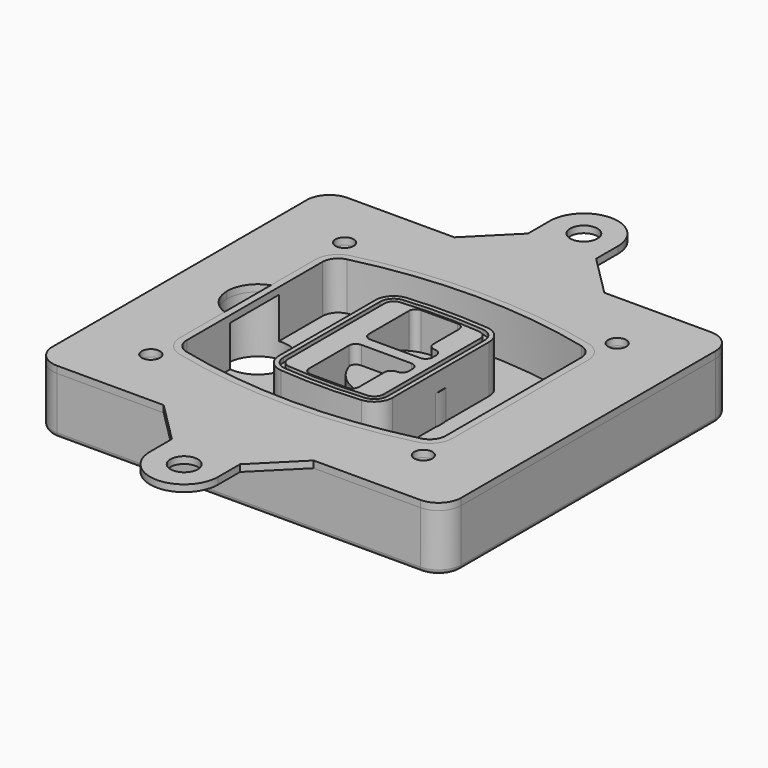
from build123d import *

# Parameters (mm, degrees)
F0_R      = 4
F1_DEPTH  = 25
F2_DEPTH  = 3
F3_DEPTH  = 18
F5_DEPTH  = 21
F6_DEPTH  = 2
F8_DEPTH  = 20
F9_DEPTH  = 16
F10_DEPTH = 25
F7_R      = 6
F7_R_2    = 4
F11_DEPTH = 6
F13_DEPTH = 9
F15_R     = 2
F16_R     = 6
F16_R_2   = 4
F17_DEPTH = 3


# Not quite as in the source:
# - a feature of the source that left no trace in its solid (it failed there, or was rolled back) is left out
# - a feature names something its author has since deleted; it is built from what else it names


with BuildPart() as f1:
    # F0 (on Top) → F1 (new body)
    with BuildSketch(Plane.XY):
        with BuildLine():
            ThreePointArc((-90, -70), (-87.0710678119, -77.0710678119), (-80, -80))
            Line((-80, -80), (80, -80))
            ThreePointArc((80, -80), (87.0710678119, -77.0710678119), (90, -70))
            Line((90, -70), (90, 70))
            ThreePointArc((90, 70), (87.0710678119, 77.0710678119), (80, 80))
            Line((80, 80), (-80, 80))
            ThreePointArc((-80, 80), (-87.0710678119, 77.0710678119), (-90, 70))
            Line((-90, 70), (-90, -70))
        make_face()
        with Locations((-60, -53.3333333333)):
            Circle(F0_R, mode=Mode.SUBTRACT)
        with Locations((60, -53.3333333333)):
            Circle(F0_R, mode=Mode.SUBTRACT)
        with Locations((-60, 53.3333333333)):
            Circle(F0_R, mode=Mode.SUBTRACT)
        with BuildLine():
            ThreePointArc((-64, 37.2990447398), (-61.0143011354, 45.9411029726), (-53.3306899286, 50.8970778549))
            ThreePointArc((-53.3306899286, 50.8970778549), (0, 57.3333333333), (53.3306899286, 50.8970778549))
            ThreePointArc((53.3306899286, 50.8970778549), (61.0143011354, 45.9411029726), (64, 37.2990447398))
            Line((64, 37.2990447398), (64, -37.2990447398))
            ThreePointArc((64, -37.2990447398), (61.0143011354, -45.9411029726), (53.3306899286, -50.8970778549))
            ThreePointArc((53.3306899286, -50.8970778549), (0, -57.3333333333), (-53.3306899286, -50.8970778549))
            ThreePointArc((-53.3306899286, -50.8970778549), (-61.0143011354, -45.9411029726), (-64, -37.2990447398))
            Line((-64, -37.2990447398), (-64, 37.2990447398))
        make_face(mode=Mode.SUBTRACT)
        with Locations((60, 53.3333333333)):
            Circle(F0_R, mode=Mode.SUBTRACT)
        with BuildLine():
            ThreePointArc((53.3306899286, 50.8970778549), (0, 57.3333333333), (-53.3306899286, 50.8970778549))
            ThreePointArc((-53.3306899286, 50.8970778549), (-61.0143011354, 45.9411029726), (-64, 37.2990447398))
            Line((-64, 37.2990447398), (-64, -37.2990447398))
            ThreePointArc((-64, -37.2990447398), (-61.0143011354, -45.9411029726), (-53.3306899286, -50.8970778549))
            ThreePointArc((-53.3306899286, -50.8970778549), (0, -57.3333333333), (53.3306899286, -50.8970778549))
            ThreePointArc((53.3306899286, -50.8970778549), (61.0143011354, -45.9411029726), (64, -37.2990447398))
            Line((64, -37.2990447398), (64, 37.2990447398))
            ThreePointArc((64, 37.2990447398), (61.0143011354, 45.9411029726), (53.3306899286, 50.8970778549))
        make_face()
        with BuildLine():
            Line((-60, -37.2990447398), (-60, 37.2990447398))
            ThreePointArc((-60, 37.2990447398), (-57.8673579538, 43.4719434775), (-52.3790642347, 47.0119255363))
            ThreePointArc((-52.3790642347, 47.0119255363), (0, 53.3333333333), (52.3790642347, 47.0119255363))
            ThreePointArc((52.3790642347, 47.0119255363), (57.8673579538, 43.4719434775), (60, 37.2990447398))
            Line((60, 37.2990447398), (60, -37.2990447398))
            ThreePointArc((60, -37.2990447398), (57.8673579538, -43.4719434775), (52.3790642347, -47.0119255363))
            ThreePointArc((52.3790642347, -47.0119255363), (0, -53.3333333333), (-52.3790642347, -47.0119255363))
            ThreePointArc((-52.3790642347, -47.0119255363), (-57.8673579538, -43.4719434775), (-60, -37.2990447398))
        make_face(mode=Mode.SUBTRACT)
        with BuildLine():
            ThreePointArc((-52.3790642347, 47.0119255363), (-57.8673579538, 43.4719434775), (-60, 37.2990447398))
            Line((-60, 37.2990447398), (-60, -37.2990447398))
            ThreePointArc((-60, -37.2990447398), (-57.8673579538, -43.4719434775), (-52.3790642347, -47.0119255363))
            ThreePointArc((-52.3790642347, -47.0119255363), (0, -53.3333333333), (52.3790642347, -47.0119255363))
            ThreePointArc((52.3790642347, -47.0119255363), (57.8673579538, -43.4719434775), (60, -37.2990447398))
            Line((60, -37.2990447398), (60, 37.2990447398))
            ThreePointArc((60, 37.2990447398), (57.8673579538, 43.4719434775), (52.3790642347, 47.0119255363))
            ThreePointArc((52.3790642347, 47.0119255363), (0, 53.3333333333), (-52.3790642347, 47.0119255363))
        make_face()
        with BuildLine():
            ThreePointArc((51.6653449643, 44.0980612973), (55.5071505677, 41.6200738562), (57, 37.2990447398))
            Line((57, 37.2990447398), (57, -37.2990447398))
            ThreePointArc((57, -37.2990447398), (55.5071505677, -41.6200738562), (51.6653449643, -44.0980612973))
            ThreePointArc((51.6653449643, -44.0980612973), (0, -50.3333333333), (-51.6653449643, -44.0980612973))
            ThreePointArc((-51.6653449643, -44.0980612973), (-55.5071505677, -41.6200738562), (-57, -37.2990447398))
            Line((-57, -37.2990447398), (-57, 37.2990447398))
            ThreePointArc((-57, 37.2990447398), (-55.5071505677, 41.6200738562), (-51.6653449643, 44.0980612973))
            ThreePointArc((-51.6653449643, 44.0980612973), (0, 50.3333333333), (51.6653449643, 44.0980612973))
        make_face(mode=Mode.SUBTRACT)
        with BuildLine():
            Line((57, -37.2990447398), (57, 37.2990447398))
            ThreePointArc((57, 37.2990447398), (55.5071505677, 41.6200738562), (51.6653449643, 44.0980612973))
            ThreePointArc((51.6653449643, 44.0980612973), (0, 50.3333333333), (-51.6653449643, 44.0980612973))
            ThreePointArc((-51.6653449643, 44.0980612973), (-55.5071505677, 41.6200738562), (-57, 37.2990447398))
            Line((-57, 37.2990447398), (-57, -37.2990447398))
            ThreePointArc((-57, -37.2990447398), (-55.5071505677, -41.6200738562), (-51.6653449643, -44.0980612973))
            ThreePointArc((-51.6653449643, -44.0980612973), (0, -50.3333333333), (51.6653449643, -44.0980612973))
            ThreePointArc((51.6653449643, -44.0980612973), (55.5071505677, -41.6200738562), (57, -37.2990447398))
        make_face()
    extrude(amount=-F1_DEPTH)

    # F0 (on Top) → F2 (join)
    with BuildSketch(Plane.XY):
        with BuildLine():
            ThreePointArc((-52.3790642347, 47.0119255363), (-57.8673579538, 43.4719434775), (-60, 37.2990447398))
            Line((-60, 37.2990447398), (-60, -37.2990447398))
            ThreePointArc((-60, -37.2990447398), (-57.8673579538, -43.4719434775), (-52.3790642347, -47.0119255363))
            ThreePointArc((-52.3790642347, -47.0119255363), (0, -53.3333333333), (52.3790642347, -47.0119255363))
            ThreePointArc((52.3790642347, -47.0119255363), (57.8673579538, -43.4719434775), (60, -37.2990447398))
            Line((60, -37.2990447398), (60, 37.2990447398))
            ThreePointArc((60, 37.2990447398), (57.8673579538, 43.4719434775), (52.3790642347, 47.0119255363))
            ThreePointArc((52.3790642347, 47.0119255363), (0, 53.3333333333), (-52.3790642347, 47.0119255363))
        make_face()
        with BuildLine():
            ThreePointArc((51.6653449643, 44.0980612973), (55.5071505677, 41.6200738562), (57, 37.2990447398))
            Line((57, 37.2990447398), (57, -37.2990447398))
            ThreePointArc((57, -37.2990447398), (55.5071505677, -41.6200738562), (51.6653449643, -44.0980612973))
            ThreePointArc((51.6653449643, -44.0980612973), (0, -50.3333333333), (-51.6653449643, -44.0980612973))
            ThreePointArc((-51.6653449643, -44.0980612973), (-55.5071505677, -41.6200738562), (-57, -37.2990447398))
            Line((-57, -37.2990447398), (-57, 37.2990447398))
            ThreePointArc((-57, 37.2990447398), (-55.5071505677, 41.6200738562), (-51.6653449643, 44.0980612973))
            ThreePointArc((-51.6653449643, 44.0980612973), (0, 50.3333333333), (51.6653449643, 44.0980612973))
        make_face(mode=Mode.SUBTRACT)
    extrude(amount=F2_DEPTH)

    # F0 (on Top) → F3 (cut)
    with BuildSketch(Plane.XY):
        with BuildLine():
            Line((57, -37.2990447398), (57, 37.2990447398))
            ThreePointArc((57, 37.2990447398), (55.5071505677, 41.6200738562), (51.6653449643, 44.0980612973))
            ThreePointArc((51.6653449643, 44.0980612973), (0, 50.3333333333), (-51.6653449643, 44.0980612973))
            ThreePointArc((-51.6653449643, 44.0980612973), (-55.5071505677, 41.6200738562), (-57, 37.2990447398))
            Line((-57, 37.2990447398), (-57, -37.2990447398))
            ThreePointArc((-57, -37.2990447398), (-55.5071505677, -41.6200738562), (-51.6653449643, -44.0980612973))
            ThreePointArc((-51.6653449643, -44.0980612973), (0, -50.3333333333), (51.6653449643, -44.0980612973))
            ThreePointArc((51.6653449643, -44.0980612973), (55.5071505677, -41.6200738562), (57, -37.2990447398))
        make_face()
    extrude(amount=-F3_DEPTH, mode=Mode.SUBTRACT)

    # F4 (on face) → F5 (join, through all)
    with BuildSketch(Plane.XY.offset(3)):
        with BuildLine():
            ThreePointArc((-25, -26.587695628), (-22.8992979869, -31.9912392117), (-17.7004291845, -34.5569740744))
            ThreePointArc((-17.7004291845, -34.5569740744), (0, -35.3333333333), (17.7004291845, -34.5569740744))
            ThreePointArc((17.7004291845, -34.5569740744), (22.8992979869, -31.9912392117), (25, -26.587695628))
            Line((25, -26.587695628), (25, 26.587695628))
            ThreePointArc((25, 26.587695628), (22.8992979869, 31.9912392117), (17.7004291845, 34.5569740744))
            ThreePointArc((17.7004291845, 34.5569740744), (0, 35.3333333333), (-17.7004291845, 34.5569740744))
            ThreePointArc((-17.7004291845, 34.5569740744), (-22.8992979869, 31.9912392117), (-25, 26.587695628))
            Line((-25, 26.587695628), (-25, -26.587695628))
        make_face()
        with BuildLine():
            ThreePointArc((17.5253218884, 32.5646544628), (21.4244734902, 30.6403533158), (23, 26.587695628))
            Line((23, 26.587695628), (23, -26.587695628))
            ThreePointArc((23, -26.587695628), (21.4244734902, -30.6403533158), (17.5253218884, -32.5646544628))
            ThreePointArc((17.5253218884, -32.5646544628), (0, -33.3333333333), (-17.5253218884, -32.5646544628))
            ThreePointArc((-17.5253218884, -32.5646544628), (-21.4244734902, -30.6403533158), (-23, -26.587695628))
            Line((-23, -26.587695628), (-23, 26.587695628))
            ThreePointArc((-23, 26.587695628), (-21.4244734902, 30.6403533158), (-17.5253218884, 32.5646544628))
            ThreePointArc((-17.5253218884, 32.5646544628), (0, 33.3333333333), (17.5253218884, 32.5646544628))
        make_face(mode=Mode.SUBTRACT)
        with BuildLine():
            Line((23, -26.587695628), (23, 26.587695628))
            ThreePointArc((23, 26.587695628), (21.4244734902, 30.6403533158), (17.5253218884, 32.5646544628))
            ThreePointArc((17.5253218884, 32.5646544628), (0, 33.3333333333), (-17.5253218884, 32.5646544628))
            ThreePointArc((-17.5253218884, 32.5646544628), (-21.4244734902, 30.6403533158), (-23, 26.587695628))
            Line((-23, 26.587695628), (-23, -26.587695628))
            ThreePointArc((-23, -26.587695628), (-21.4244734902, -30.6403533158), (-17.5253218884, -32.5646544628))
            ThreePointArc((-17.5253218884, -32.5646544628), (0, -33.3333333333), (17.5253218884, -32.5646544628))
            ThreePointArc((17.5253218884, -32.5646544628), (21.4244734902, -30.6403533158), (23, -26.587695628))
        make_face()
        with BuildLine():
            ThreePointArc((17.3502145923, 30.5723348512), (19.9496489934, 29.2894674198), (21, 26.587695628))
            Line((21, 26.587695628), (21, -26.587695628))
            ThreePointArc((21, -26.587695628), (19.9496489934, -29.2894674198), (17.3502145923, -30.5723348512))
            ThreePointArc((17.3502145923, -30.5723348512), (0, -31.3333333333), (-17.3502145923, -30.5723348512))
            ThreePointArc((-17.3502145923, -30.5723348512), (-19.9496489934, -29.2894674198), (-21, -26.587695628))
            Line((-21, -26.587695628), (-21, 26.587695628))
            ThreePointArc((-21, 26.587695628), (-19.9496489934, 29.2894674198), (-17.3502145923, 30.5723348512))
            ThreePointArc((-17.3502145923, 30.5723348512), (0, 31.3333333333), (17.3502145923, 30.5723348512))
        make_face(mode=Mode.SUBTRACT)
        with BuildLine():
            Line((21, -26.587695628), (21, 26.587695628))
            ThreePointArc((21, 26.587695628), (19.9496489934, 29.2894674198), (17.3502145923, 30.5723348512))
            ThreePointArc((17.3502145923, 30.5723348512), (0, 31.3333333333), (-17.3502145923, 30.5723348512))
            ThreePointArc((-17.3502145923, 30.5723348512), (-19.9496489934, 29.2894674198), (-21, 26.587695628))
            Line((-21, 26.587695628), (-21, -26.587695628))
            ThreePointArc((-21, -26.587695628), (-19.9496489934, -29.2894674198), (-17.3502145923, -30.5723348512))
            ThreePointArc((-17.3502145923, -30.5723348512), (0, -31.3333333333), (17.3502145923, -30.5723348512))
            ThreePointArc((17.3502145923, -30.5723348512), (19.9496489934, -29.2894674198), (21, -26.587695628))
        make_face()
        with BuildLine():
            Line((-8, -2.5), (14, -2.5))
            ThreePointArc((14, -2.5), (16.1213203436, -3.3786796564), (17, -5.5))
            Line((17, -5.5), (17, -7.5))
            ThreePointArc((17, -7.5), (16.1213203436, -9.6213203436), (14, -10.5))
            ThreePointArc((14, -10.5), (11.8786796564, -11.3786796564), (11, -13.5))
            Line((11, -13.5), (11, -27.5))
            ThreePointArc((11, -27.5), (10.1213203436, -29.6213203436), (8, -30.5))
            Line((8, -30.5), (-8, -30.5))
            ThreePointArc((-8, -30.5), (-10.1213203436, -29.6213203436), (-11, -27.5))
            Line((-11, -27.5), (-11, -5.5))
            ThreePointArc((-11, -5.5), (-10.1213203436, -3.3786796564), (-8, -2.5))
        make_face(mode=Mode.SUBTRACT)
        with BuildLine():
            ThreePointArc((-8, 2.5), (-10.1213203436, 3.3786796564), (-11, 5.5))
            Line((-11, 5.5), (-11, 27.5))
            ThreePointArc((-11, 27.5), (-10.1213203436, 29.6213203436), (-8, 30.5))
            Line((-8, 30.5), (8, 30.5))
            ThreePointArc((8, 30.5), (10.1213203436, 29.6213203436), (11, 27.5))
            Line((11, 27.5), (11, 13.5))
            ThreePointArc((11, 13.5), (11.8786796564, 11.3786796564), (14, 10.5))
            ThreePointArc((14, 10.5), (16.1213203436, 9.6213203436), (17, 7.5))
            Line((17, 7.5), (17, 5.5))
            ThreePointArc((17, 5.5), (16.1213203436, 3.3786796564), (14, 2.5))
            Line((14, 2.5), (-8, 2.5))
        make_face(mode=Mode.SUBTRACT)
    extrude(amount=-F5_DEPTH)

    # F4 (on face) → F6 (cut)
    with BuildSketch(Plane.XY.offset(3)):
        with BuildLine():
            Line((23, -26.587695628), (23, 26.587695628))
            ThreePointArc((23, 26.587695628), (21.4244734902, 30.6403533158), (17.5253218884, 32.5646544628))
            ThreePointArc((17.5253218884, 32.5646544628), (0, 33.3333333333), (-17.5253218884, 32.5646544628))
            ThreePointArc((-17.5253218884, 32.5646544628), (-21.4244734902, 30.6403533158), (-23, 26.587695628))
            Line((-23, 26.587695628), (-23, -26.587695628))
            ThreePointArc((-23, -26.587695628), (-21.4244734902, -30.6403533158), (-17.5253218884, -32.5646544628))
            ThreePointArc((-17.5253218884, -32.5646544628), (0, -33.3333333333), (17.5253218884, -32.5646544628))
            ThreePointArc((17.5253218884, -32.5646544628), (21.4244734902, -30.6403533158), (23, -26.587695628))
        make_face()
        with BuildLine():
            ThreePointArc((17.3502145923, 30.5723348512), (19.9496489934, 29.2894674198), (21, 26.587695628))
            Line((21, 26.587695628), (21, -26.587695628))
            ThreePointArc((21, -26.587695628), (19.9496489934, -29.2894674198), (17.3502145923, -30.5723348512))
            ThreePointArc((17.3502145923, -30.5723348512), (0, -31.3333333333), (-17.3502145923, -30.5723348512))
            ThreePointArc((-17.3502145923, -30.5723348512), (-19.9496489934, -29.2894674198), (-21, -26.587695628))
            Line((-21, -26.587695628), (-21, 26.587695628))
            ThreePointArc((-21, 26.587695628), (-19.9496489934, 29.2894674198), (-17.3502145923, 30.5723348512))
            ThreePointArc((-17.3502145923, 30.5723348512), (0, 31.3333333333), (17.3502145923, 30.5723348512))
        make_face(mode=Mode.SUBTRACT)
    extrude(amount=-F6_DEPTH, mode=Mode.SUBTRACT)

    # F7 (on face) → F8 (join)
    with BuildSketch(Plane(origin=(0, 0, -25), x_dir=(1, 0, 0), z_dir=(0, 0, -1))):
        with BuildLine():
            ThreePointArc((-6.71157564, 0), (6.7567035675, 13.4682792075), (20.224982775, 0))
            Line((20.224982775, 0), (25.224982775, 0))
            ThreePointArc((25.224982775, 0), (6.7567035675, 18.4682792075), (-11.71157564, 0))
            Line((-11.71157564, 0), (-6.71157564, 0))
        make_face()
        with BuildLine():
            Line((-6.71157564, 0), (20.224982775, 0))
            ThreePointArc((20.224982775, 0), (6.7567035675, 13.4682792075), (-6.71157564, 0))
        make_face()
        with BuildLine():
            ThreePointArc((-6.71157564, 0), (6.7567035675, -13.4682792075), (20.224982775, 0))
            Line((20.224982775, 0), (-6.71157564, 0))
        make_face()
        with BuildLine():
            Line((25.224982775, 0), (20.224982775, 0))
            ThreePointArc((20.224982775, 0), (6.7567035675, -13.4682792075), (-6.71157564, 0))
            Line((-6.71157564, 0), (-11.71157564, 0))
            ThreePointArc((-11.71157564, 0), (6.7567035675, -18.4682792075), (25.224982775, 0))
        make_face()
    extrude(amount=-F8_DEPTH)

    # F7 (on face) → F9 (cut)
    with BuildSketch(Plane(origin=(0, 0, -25), x_dir=(1, 0, 0), z_dir=(0, 0, -1))):
        with BuildLine():
            Line((-6.71157564, 0), (20.224982775, 0))
            ThreePointArc((20.224982775, 0), (6.7567035675, 13.4682792075), (-6.71157564, 0))
        make_face()
        with BuildLine():
            ThreePointArc((-6.71157564, 0), (6.7567035675, -13.4682792075), (20.224982775, 0))
            Line((20.224982775, 0), (-6.71157564, 0))
        make_face()
    extrude(amount=-F9_DEPTH, mode=Mode.SUBTRACT)

    # F7 (on face) → F10 (cut)
    with BuildSketch(Plane(origin=(0, 0, -25), x_dir=(1, 0, 0), z_dir=(0, 0, -1))):
        with BuildLine():
            Line((-69.0318229325, 0), (-42.0952645175, 0))
            ThreePointArc((-42.0952645175, 0), (-55.563543725, 13.4682792075), (-69.0318229325, 0))
        make_face()
        with BuildLine():
            ThreePointArc((-69.0318229325, 0), (-55.563543725, -13.4682792075), (-42.0952645175, 0))
            Line((-42.0952645175, 0), (-69.0318229325, 0))
        make_face()
    extrude(amount=-F10_DEPTH, mode=Mode.SUBTRACT)

    # F7 (on face) → F11 (cut)
    with BuildSketch(Plane(origin=(0, 0, -25), x_dir=(1, 0, 0), z_dir=(0, 0, -1))):
        with Locations((60, -53.3333333333)):
            Circle(F7_R)
        with Locations((60, -53.3333333333)):
            Circle(F7_R_2, mode=Mode.SUBTRACT)
        with Locations((-60, -53.3333333333)):
            Circle(F7_R)
        with Locations((-60, -53.3333333333)):
            Circle(F7_R_2, mode=Mode.SUBTRACT)
        with Locations((-60, 53.3333333333)):
            Circle(F7_R)
        with Locations((-60, 53.3333333333)):
            Circle(F7_R_2, mode=Mode.SUBTRACT)
        with Locations((60, 53.3333333333)):
            Circle(F7_R)
        with Locations((60, 53.3333333333)):
            Circle(F7_R_2, mode=Mode.SUBTRACT)
    extrude(amount=-F11_DEPTH, mode=Mode.SUBTRACT)

    # F12 (on face) → F13 (cut, through all)
    with BuildSketch(Plane(origin=(0, 0, -9), x_dir=(1, 0, 0), z_dir=(0, 0, -1))):
        with BuildLine():
            ThreePointArc((20.224982775, 0), (20.1663399806, 1.2554664788), (19.9909222755, 2.5))
            Line((19.9909222755, 2.5), (14, 2.5))
            ThreePointArc((14, 2.5), (16.1213203436, 3.3786796564), (17, 5.5))
            Line((17, 5.5), (17, 7.5))
            ThreePointArc((17, 7.5), (16.1213203436, 9.6213203436), (14, 10.5))
            ThreePointArc((14, 10.5), (12.1627255951, 11.1284134507), (11.0951631559, 12.750384826))
            ThreePointArc((11.0951631559, 12.750384826), (11.0476113807, 12.7664660322), (11, 12.7823698976))
            Line((11, 12.7823698976), (11, -12.7823698976))
            ThreePointArc((11, -12.7823698976), (11.0476113807, -12.7664660322), (11.0951631559, -12.750384826))
            ThreePointArc((11.0951631559, -12.750384826), (12.1627255951, -11.1284134507), (14, -10.5))
            ThreePointArc((14, -10.5), (16.1213203436, -9.6213203436), (17, -7.5))
            Line((17, -7.5), (17, -5.5))
            ThreePointArc((17, -5.5), (16.1213203436, -3.3786796564), (14, -2.5))
            Line((14, -2.5), (19.9909222755, -2.5))
            ThreePointArc((19.9909222755, -2.5), (20.1663399806, -1.2554664788), (20.224982775, 0))
        make_face()
    extrude(amount=F13_DEPTH, mode=Mode.SUBTRACT)

    # F15
    f15_edges = [f1.edges().sort_by_distance(p)[0] for p in [
        (0, -80, -25),
        (-87.071068, -77.071068, -25),
        (-90, 0, -25),
        (-87.071068, 77.071068, -25),
        (87.071068, -77.071068, -25),
        (0, 80, -25),
        (90, 0, -25),
        (87.071068, 77.071068, -25),
    ]]
    fillet(f15_edges, radius=F15_R)


with BuildPart() as f17:
    # F16 (on face) → F17 (new body, through all)
    with BuildSketch(Plane.XY):
        with BuildLine():
            Line((-15, 98), (-33, 80))
            Line((-33, 80), (33, 80))
            Line((33, 80), (15, 98))
            Line((15, 98), (15, 110))
            ThreePointArc((15, 110), (0, 125), (-15, 110))
            Line((-15, 110), (-15, 98))
        make_face()
        with Locations((0, 110)):
            Circle(F16_R, mode=Mode.SUBTRACT)
        with BuildLine():
            Line((-33, 80), (-80, 80))
            ThreePointArc((-80, 80), (-87.0710678119, 77.0710678119), (-90, 70))
            Line((-90, 70), (-90, -70))
            ThreePointArc((-90, -70), (-87.0710678119, -77.0710678119), (-80, -80))
            Line((-80, -80), (-33, -80))
            Line((-33, -80), (33, -80))
            Line((33, -80), (80, -80))
            ThreePointArc((80, -80), (87.0710678119, -77.0710678119), (90, -70))
            Line((90, -70), (90, 70))
            ThreePointArc((90, 70), (87.0710678119, 77.0710678119), (80, 80))
            Line((80, 80), (33, 80))
            Line((33, 80), (-33, 80))
        make_face()
        with Locations((-60, -53.3333333333)):
            Circle(F16_R_2, mode=Mode.SUBTRACT)
        with BuildLine():
            ThreePointArc((-60, 37.2990447398), (-57.8673579538, 43.4719434775), (-52.3790642347, 47.0119255363))
            ThreePointArc((-52.3790642347, 47.0119255363), (0, 53.3333333333), (52.3790642347, 47.0119255363))
            ThreePointArc((52.3790642347, 47.0119255363), (57.8673579538, 43.4719434775), (60, 37.2990447398))
            Line((60, 37.2990447398), (60, -37.2990447398))
            ThreePointArc((60, -37.2990447398), (57.8673579538, -43.4719434775), (52.3790642347, -47.0119255363))
            ThreePointArc((52.3790642347, -47.0119255363), (0, -53.3333333333), (-52.3790642347, -47.0119255363))
            ThreePointArc((-52.3790642347, -47.0119255363), (-57.8673579538, -43.4719434775), (-60, -37.2990447398))
            Line((-60, -37.2990447398), (-60, -12.7166190685))
            ThreePointArc((-60, -12.7166190685), (-66.5441169481, -7.798817635), (-69.0318229325, 0))
            ThreePointArc((-69.0318229325, 0), (-66.5441169481, 7.798817635), (-60, 12.7166190685))
            Line((-60, 12.7166190685), (-60, 37.2990447398))
        make_face(mode=Mode.SUBTRACT)
        with Locations((60, -53.3333333333)):
            Circle(F16_R_2, mode=Mode.SUBTRACT)
        with Locations((-60, 53.3333333333)):
            Circle(F16_R_2, mode=Mode.SUBTRACT)
        with Locations((60, 53.3333333333)):
            Circle(F16_R_2, mode=Mode.SUBTRACT)
        with BuildLine():
            Line((33, -80), (-33, -80))
            Line((-33, -80), (-15, -98))
            Line((-15, -98), (-15, -110))
            ThreePointArc((-15, -110), (0, -125), (15, -110))
            Line((15, -110), (15, -98))
            Line((15, -98), (33, -80))
        make_face()
        with Locations((0, -110)):
            Circle(F16_R, mode=Mode.SUBTRACT)
    extrude(amount=F17_DEPTH)


solid = Compound([f1.part, f17.part])
